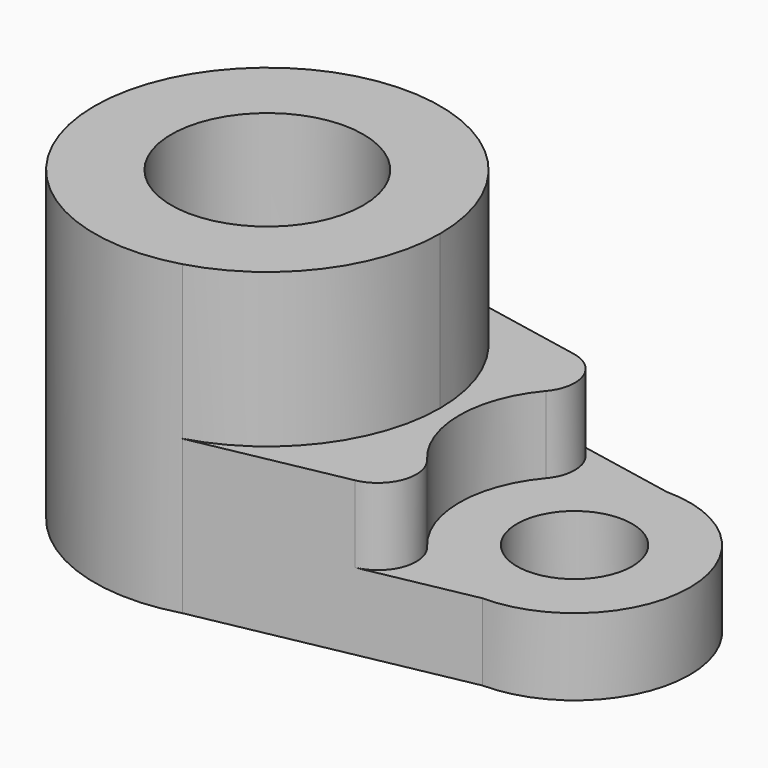
from build123d import *

# Parameters (mm, degrees)
F0_R     = 15.875
F0_R_2   = 9.525
F1_DEPTH = 25.4
F2_DEPTH = 25.4
F3_DEPTH = 12.7
F4_R     = 6.35


with BuildPart() as f1:
    # F0 (on Top) → F1 (new body)
    with BuildSketch(Plane.XY):
        with BuildLine():
            ThreePointArc((7.9032867525, -27.4603110599), (22.829444189, -17.1856656264), (28.575, 0))
            ThreePointArc((28.575, 0), (22.829444189, 17.1856656264), (7.9032867525, 27.4603110599))
            ThreePointArc((7.9032867525, 27.4603110599), (-28.575, 0), (7.9032867525, -27.4603110599))
        make_face()
        Circle(F0_R, mode=Mode.SUBTRACT)
        with BuildLine():
            ThreePointArc((7.9032867525, 27.4603110599), (22.829444189, 17.1856656264), (28.575, 0))
            ThreePointArc((28.575, 0), (22.829444189, -17.1856656264), (7.9032867525, -27.4603110599))
            Line((7.9032867525, -27.4603110599), (50.8, -19.05))
            ThreePointArc((50.8, -19.05), (31.75, 0), (50.8, 19.05))
            Line((50.8, 19.05), (7.9032867525, 27.4603110599))
        make_face()
        with BuildLine():
            ThreePointArc((69.85, 0), (64.2703841816, 13.4703841816), (50.8, 19.05))
            ThreePointArc((50.8, 19.05), (31.75, 0), (50.8, -19.05))
            ThreePointArc((50.8, -19.05), (64.2703841816, -13.4703841816), (69.85, 0))
        make_face()
        with Locations((50.8, 0)):
            Circle(F0_R_2, mode=Mode.SUBTRACT)
    extrude(amount=-F1_DEPTH)

    # F0 (on Top) → F2 (join)
    with BuildSketch(Plane.XY):
        with BuildLine():
            ThreePointArc((7.9032867525, -27.4603110599), (22.829444189, -17.1856656264), (28.575, 0))
            ThreePointArc((28.575, 0), (22.829444189, 17.1856656264), (7.9032867525, 27.4603110599))
            ThreePointArc((7.9032867525, 27.4603110599), (-28.575, 0), (7.9032867525, -27.4603110599))
        make_face()
        Circle(F0_R, mode=Mode.SUBTRACT)
    extrude(amount=F2_DEPTH)

    # F0 (on Top) → F3 (cut)
    with BuildSketch(Plane.XY):
        with BuildLine():
            ThreePointArc((69.85, 0), (64.2703841816, 13.4703841816), (50.8, 19.05))
            ThreePointArc((50.8, 19.05), (31.75, 0), (50.8, -19.05))
            ThreePointArc((50.8, -19.05), (64.2703841816, -13.4703841816), (69.85, 0))
        make_face()
        with Locations((50.8, 0)):
            Circle(F0_R_2, mode=Mode.SUBTRACT)
    extrude(amount=-F3_DEPTH, mode=Mode.SUBTRACT)

    # F4
    f4_edges = [f1.edges().sort_by_distance(p)[0] for p in [
        (50.8, 19.05, -6.35),
        (50.8, -19.05, -6.35),
    ]]
    fillet(f4_edges, radius=F4_R)


solid = f1.part
